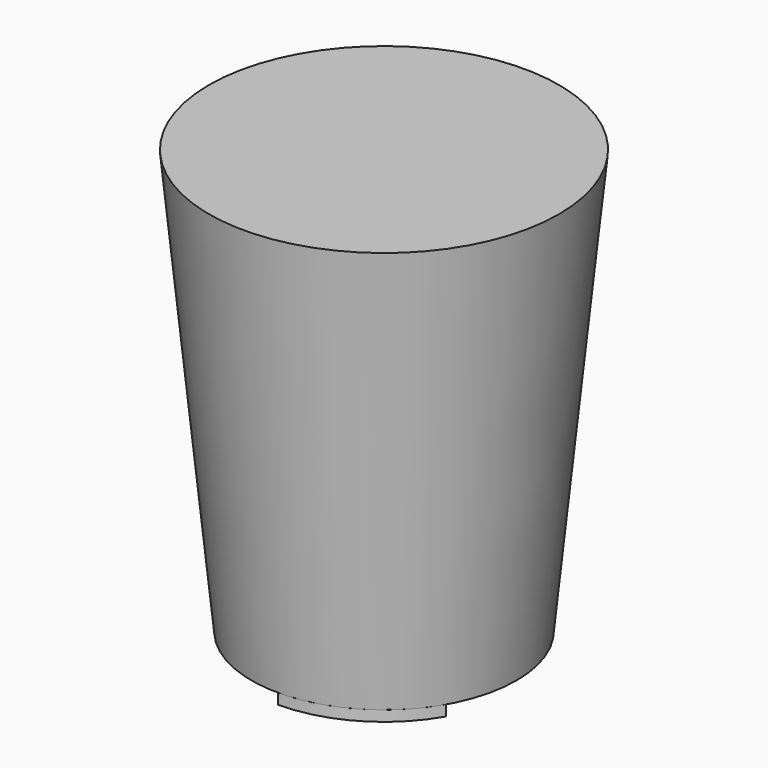
from build123d import *

# Parameters (mm, degrees)
F2_R     = 25
F3_R     = 33
F5_R     = 5
F6_DEPTH = 0.6
F8_DEPTH = 2


# Not quite as in the source:
# - a feature names something its author has since deleted; it is built from what else it names


with BuildPart() as f4:
    # F2 (on Top) → F4 section 0
    with BuildSketch(Plane.XY):
        Circle(F2_R)
    # F3 (on offset) → F4 section 1
    with BuildSketch(Plane.XY.offset(80)):
        Circle(F3_R)
    loft()

    # F5 (on face) → F6 (cut)
    with BuildSketch(Plane(origin=(0, 0, 0), x_dir=(1, 0, 0), z_dir=(0, 0, -1))):
        Circle(F5_R)
    extrude(amount=-F6_DEPTH, mode=Mode.SUBTRACT)


with BuildPart() as f8:
    # F7 (on face) → F8 (new body)
    with BuildSketch(Plane(origin=(0, 0, 0), x_dir=(1, 0, 0), z_dir=(0, 0, -1))):
        with BuildLine():
            ThreePointArc((21.6506350946, 12.5), (12.5, 21.6506350946), (0, 25))
            Line((0, 25), (0, 22))
            ThreePointArc((0, 22), (11, 19.0525588833), (19.0525588833, 11))
            Line((19.0525588833, 11), (21.6506350946, 12.5))
        make_face()
    extrude(amount=F8_DEPTH)


solid = Compound([f4.part, f8.part])
